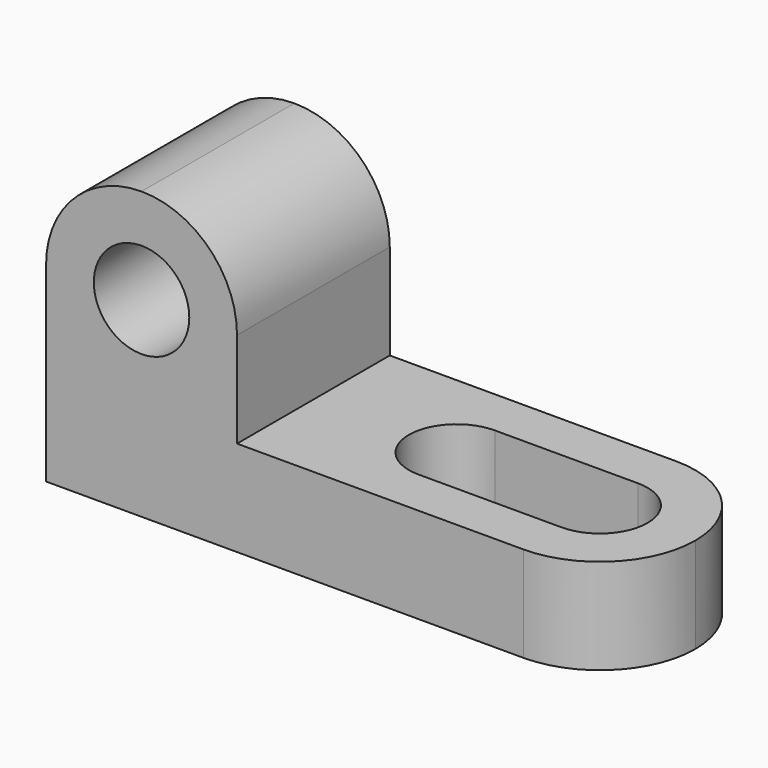
from build123d import *

# Parameters (mm, degrees)
F1_DEPTH = 25.4
F2_R     = 12.69999
F3_R     = 6.35
F4_DEPTH = 25.4
F6_DEPTH = 25.4


# Not quite as in the source:
# - a fillet or chamfer is up to 0.001 mm smaller than in the source, because OpenCascade refuses the exact size


with BuildPart() as f1:
    # F0 (on Front) → F1 (new body)
    with BuildSketch(Plane.XZ):
        Polygon((0, 38.1), (0, 0), (76.2, 0), (76.2, 12.7), (25.4, 12.7), (25.4, 38.1), align=None)
    extrude(amount=F1_DEPTH)

    # F2 (radius 12.7 in the source; OpenCascade refuses exactly that, so slightly less here)
    f2_edges = [f1.edges().sort_by_distance(p)[0] for p in [
        (25.4, -12.7, 38.1),
        (0, -12.7, 38.1),
        (76.2, -25.4, 6.35),
        (76.2, 0, 6.35),
    ]]
    fillet(f2_edges, radius=F2_R)

    # F3 (on face) → F4 (cut)
    with BuildSketch(Plane.XZ.offset(25.4)):
        with Locations((12.7, 25.4)):
            Circle(F3_R)
    extrude(amount=-F4_DEPTH, mode=Mode.SUBTRACT)

    # F5 (on face) → F6 (cut)
    with BuildSketch(Plane.XY.offset(12.7)):
        with BuildLine():
            ThreePointArc((44.45, -19.05), (48.9401287414, -17.1901284329), (50.8000010533, -12.7))
            ThreePointArc((50.8000010533, -12.7), (48.9401287414, -8.2098715671), (44.45, -6.35))
            ThreePointArc((44.45, -6.35), (38.1000010533, -12.7), (44.45, -19.05))
        make_face()
        with BuildLine():
            ThreePointArc((44.45, -6.35), (48.9401287414, -8.2098715671), (50.8000010533, -12.7))
            ThreePointArc((50.8000010533, -12.7), (48.9401287414, -17.1901284329), (44.45, -19.05))
            Line((44.45, -19.05), (63.5, -19.05))
            ThreePointArc((63.5, -19.05), (57.15, -12.7), (63.5, -6.35))
            Line((63.5, -6.35), (44.45, -6.35))
        make_face()
        with BuildLine():
            ThreePointArc((69.85, -12.7), (67.9901280605, -8.2098719395), (63.5, -6.35))
            ThreePointArc((63.5, -6.35), (57.15, -12.7), (63.5, -19.05))
            ThreePointArc((63.5, -19.05), (67.9901280605, -17.1901280605), (69.85, -12.7))
        make_face()
    extrude(amount=-F6_DEPTH, mode=Mode.SUBTRACT)


solid = f1.part
